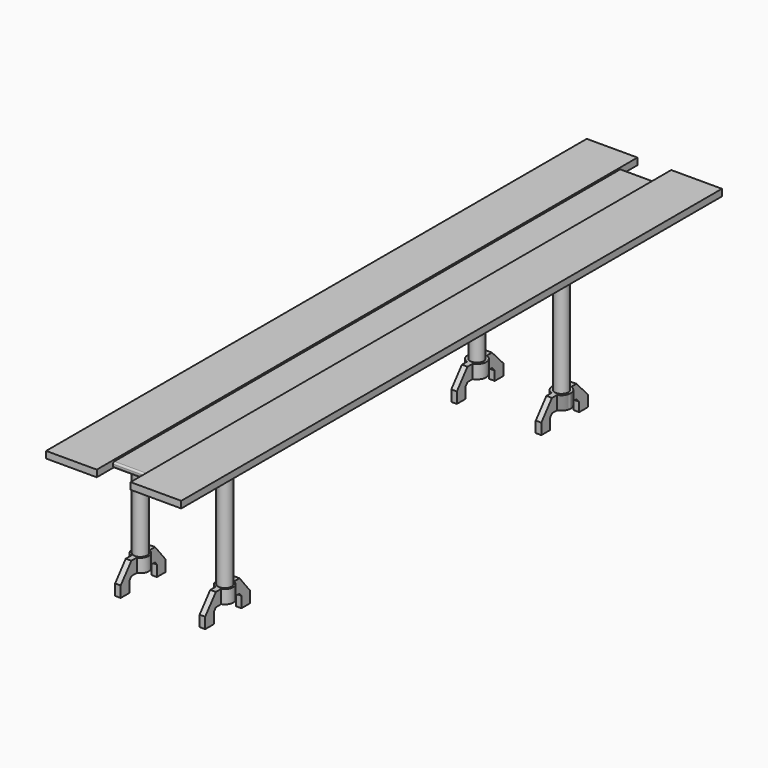
from build123d import *

# Parameters (mm, degrees)
F1_DEPTH  = 4000
F2_W      = 200
F2_H      = 120
F3_DEPTH  = 55.88
F4_R      = 10
F5_R      = 55
F5_R_2    = 40
F6_DEPTH  = 80
F7_W      = 5
F7_H      = 50
F8_DEPTH  = 80
F10_DEPTH = 605.001
F11_R     = 40
F12_DEPTH = 730
F13_R     = 50
F13_R_2   = 40
F14_DEPTH = 80
F17_DEPTH = 16.5
F19_R     = 55
F19_R_2   = 40
F20_DEPTH = 80
F24_DEPTH = 16.5
F26_W     = 5
F26_H     = 80
F27_DEPTH = 25.4
F28_W     = 80
F28_H     = 5
F29_DEPTH = 25.4
F30_W     = 80
F30_H     = 5
F31_DEPTH = 25.4


# Not quite as in the source:
# - ends of sketch curves that miss each other by under 0.0002 mm in the source are joined


with BuildPart() as f1:
    # F0 (on Front) → F1 (new body)
    with BuildSketch(Plane.XZ):
        Polygon((-100, 10), (-100, 20), (-400, 20), (-400, -20), (400, -20), (400, 20), (100, 20), (100, 10), align=None)
    extrude(amount=-F1_DEPTH)

    # F2 (on face) → F3 (cut)
    with BuildSketch(Plane.XY.offset(10)):
        with Locations((0, 60)):
            Rectangle(F2_W, F2_H)
        with Locations((0, 3940)):
            Rectangle(F2_W, F2_H)
    extrude(amount=-F3_DEPTH, mode=Mode.SUBTRACT)

    # F4
    f4_edges = [f1.edges().sort_by_distance(p)[0] for p in [
        (0, 3880, 10),
        (0, 120, 10),
        (0, 120, -20),
        (0, 3880, -20),
    ]]
    fillet(f4_edges, radius=F4_R)

    # F5 (on face) → F6 (join)
    with BuildSketch(Plane(origin=(0, 0, -20), x_dir=(1, 0, 0), z_dir=(0, 0, -1))):
        with Locations((-250, -510)):
            Circle(F5_R)
        with Locations((-250, -510)):
            Circle(F5_R_2, mode=Mode.SUBTRACT)
        with Locations((-250, -3000)):
            Circle(F5_R)
        with Locations((-250, -3000)):
            Circle(F5_R_2, mode=Mode.SUBTRACT)
        with Locations((250, -510)):
            Circle(F5_R)
        with Locations((250, -510)):
            Circle(F5_R_2, mode=Mode.SUBTRACT)
        with Locations((250, -3000)):
            Circle(F5_R)
        with Locations((250, -3000)):
            Circle(F5_R_2, mode=Mode.SUBTRACT)
    extrude(amount=F6_DEPTH)

    # F7 (on face) → F8 (join)
    with BuildSketch(Plane(origin=(0, 0, -20), x_dir=(1, 0, 0), z_dir=(0, 0, -1))):
        with Locations((-202.5, -2000)):
            Rectangle(F7_W, F7_H)
        with Locations((202.5, -2000)):
            Rectangle(F7_W, F7_H)
    extrude(amount=F8_DEPTH)

    # F9 (on face) → F10 (cut, through all)
    with BuildSketch(Plane(origin=(-205, 0, 0), x_dir=(0, -1, 0), z_dir=(-1, 0, 0))):
        with BuildLine():
            Line((-1995, -90), (-1995, -30))
            ThreePointArc((-1995, -30), (-2000, -25), (-2005, -30))
            Line((-2005, -30), (-2005, -90))
            Line((-2005, -90), (-2005, -90.002886951))
            ThreePointArc((-2005, -90.002886951), (-2000.0005923209, -94.9999999649), (-1995.0000016578, -90.0040715919))
            Line((-1995.0000016578, -90.0040715919), (-1995, -90))
        make_face()
    extrude(amount=-F10_DEPTH, mode=Mode.SUBTRACT)

    # F11 (on face) → F12 (join)
    with BuildSketch(Plane(origin=(0, 0, -20), x_dir=(1, 0, 0), z_dir=(0, 0, -1))):
        with Locations((250, -3000)):
            Circle(F11_R)
        with Locations((-250, -3000)):
            Circle(F11_R)
        with Locations((-250, -510)):
            Circle(F11_R)
        with Locations((250, -510)):
            Circle(F11_R)
    extrude(amount=F12_DEPTH)

    # F26 (on face) → F27 (join)
    with BuildSketch(Plane(origin=(0, 0, -20), x_dir=(1, 0, 0), z_dir=(0, 0, -1))):
        with Locations((142.5, -3920)):
            Rectangle(F26_W, F26_H)
        with Locations((-142.5, -3920)):
            Rectangle(F26_W, F26_H)
    extrude(amount=F27_DEPTH)

    # F28 (on face) → F29 (join)
    with BuildSketch(Plane(origin=(-145, 0, 0), x_dir=(0, -1, 0), z_dir=(-1, 0, 0))):
        with Locations((-3920, -42.9)):
            Rectangle(F28_W, F28_H)
    extrude(amount=F29_DEPTH)

    # F30 (on face) → F31 (join)
    with BuildSketch(Plane.YZ.offset(145)):
        with Locations((3920, -42.9)):
            Rectangle(F30_W, F30_H)
    extrude(amount=F31_DEPTH)


with BuildPart() as f14:
    # F13 (on face) → F14 (new body)
    with BuildSketch(Plane(origin=(0, 0, -750), x_dir=(1, 0, 0), z_dir=(0, 0, -1))):
        with Locations((-250, -510)):
            Circle(F13_R)
        with Locations((-250, -510)):
            Circle(F13_R_2, mode=Mode.SUBTRACT)
    extrude(amount=-F14_DEPTH)

    # F16 (on face) → F17 (join, symmetric)
    with BuildSketch(Plane(origin=(-250, 0, 0), x_dir=(0, -1, 0), z_dir=(-1, 0, 0))):
        Polygon((-558.1679285306, -750), (-558.1679285306, -670), (-598.1679285306, -670), (-676.9920066674, -767.0142500145), (-676.9920066674, -832.0142500145), (-611.9920066674, -832.0142500145), (-611.9920066674, -767.0142500145), (-598.1679285306, -750), align=None)
        Polygon((-422.7537339867, -670), (-462.7537339867, -670), (-462.7537339867, -750), (-422.7537339867, -750), (-408.9296558499, -767.0142500145), (-408.9296558499, -832.0142500145), (-343.9296558499, -832.0142500145), (-343.9296558499, -767.0142500145), align=None)
    extrude(amount=F17_DEPTH, both=True)


with BuildPart() as f18_1:
    # F18: instance of F14
    add(f14.part.mirror(Plane.YZ))


with BuildPart() as f20:
    # F19 (on face) → F20 (new body)
    with BuildSketch(Plane(origin=(0, 0, -750), x_dir=(1, 0, 0), z_dir=(0, 0, -1))):
        with Locations((-250, -3000)):
            Circle(F19_R)
        with Locations((-250, -3000)):
            Circle(F19_R_2, mode=Mode.SUBTRACT)
    extrude(amount=-F20_DEPTH)


with BuildPart() as f21_1:
    # F21: instance of F20
    add(f20.part.mirror(Plane.YZ))


with BuildPart() as f20_1:
    add(f20.part)

    # F23 (on face) → F24 (join, symmetric)
    with BuildSketch(Plane(origin=(-250, 0, 0), x_dir=(0, -1, 0), z_dir=(-1, 0, 0))):
        Polygon((-2909.501227852, -670), (-2949.501227852, -670), (-2949.501227852, -750), (-2909.501227852, -750), (-2895.6771497151, -767.0142500145), (-2895.6771497151, -832.0142500145), (-2830.6771497151, -832.0142500145), (-2830.6771497151, -767.0142500145), align=None)
        Polygon((-3050.5731344893, -750), (-3050.5731344893, -670), (-3090.5731344893, -670), (-3176.1190319061, -761.1421934954), (-3176.1190319061, -826.1421934954), (-3111.1190319061, -826.1421934954), (-3111.1190319061, -771.8899820383), (-3090.5731344893, -750), align=None)
    extrude(amount=F24_DEPTH, both=True)


with BuildPart() as f25_1:
    # F25: instance of F20
    add(f20_1.part.mirror(Plane.YZ))


solid = Compound([f1.part, f14.part, f18_1.part, f21_1.part, f20_1.part, f25_1.part])
